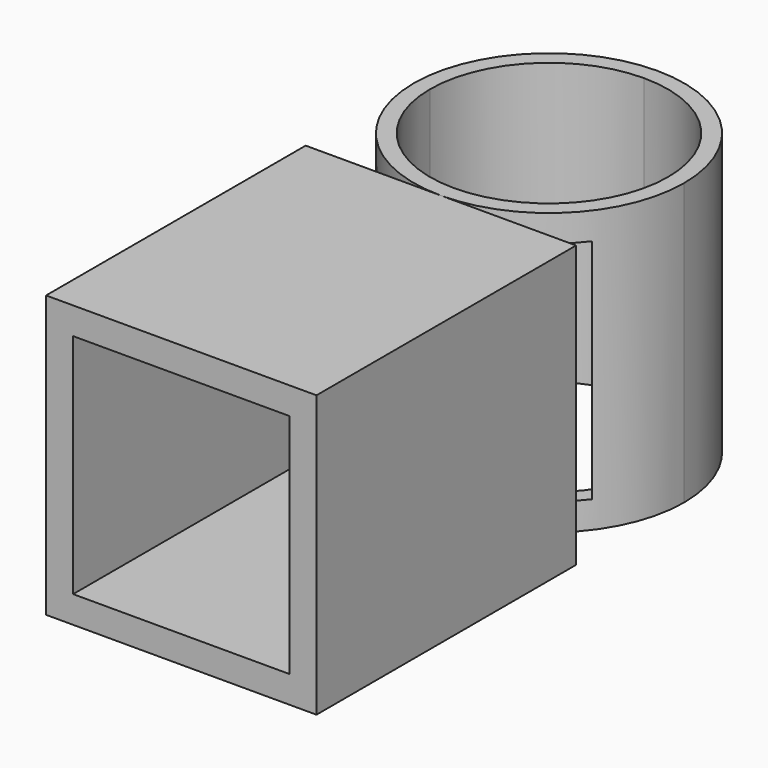
from build123d import *

# Parameters (mm, degrees)
F1_DEPTH = 26
F3_W     = 25
F3_H     = 26
F4_DEPTH = 30
F5_T     = -2.5
F6_DEPTH = 15


with BuildPart() as f1:
    # F0 (on Top) → F1 (new body)
    with BuildSketch(Plane.XY):
        with BuildLine():
            Line((11, 0), (12.5, 0))
            ThreePointArc((12.5, 0), (8.8388347648, 8.8388347648), (0, 12.5))
            Line((0, 12.5), (0, 11))
            ThreePointArc((0, 11), (7.7781745931, 7.7781745931), (11, 0))
        make_face()
        with BuildLine():
            Line((0, 11), (0, 12.5))
            ThreePointArc((0, 12.5), (-8.8388347648, 8.8388347648), (-12.5, 0))
            Line((-12.5, 0), (-11, 0))
            ThreePointArc((-11, 0), (-7.7781745931, 7.7781745931), (0, 11))
        make_face()
        with BuildLine():
            ThreePointArc((-12.5, 0), (-8.8388347648, -8.8388347648), (0, -12.5))
            Line((0, -12.5), (0, -11))
            ThreePointArc((0, -11), (-7.7781745931, -7.7781745931), (-11, 0))
            Line((-11, 0), (-12.5, 0))
        make_face()
        with BuildLine():
            ThreePointArc((0, -12.5), (8.8388347648, -8.8388347648), (12.5, 0))
            Line((12.5, 0), (11, 0))
            ThreePointArc((11, 0), (7.7781745931, -7.7781745931), (0, -11))
            Line((0, -11), (0, -12.5))
        make_face()
    extrude(amount=F1_DEPTH)


with BuildPart() as f4:
    # F3 (on offset) → F4 (new body)
    with BuildSketch(Plane.XZ.offset(12.5)):
        with Locations((-0.0008905306, 13)):
            Rectangle(F3_W, F3_H)
    extrude(amount=F4_DEPTH)

    # F5
    f5_openings = [f4.faces().sort_by_distance(p)[0] for p in [
        (-0.000891, -42.5, 13),
    ]]
    offset(amount=F5_T, openings=f5_openings)


with BuildPart() as f6_tool:
    # F6 (cut): a face of the model
    f6_faces = [f4.part.faces().sort_by_distance(p)[0] for p in [
        (-0.0008905306, -15, 13),
    ]]
    extrude(f6_faces, amount=-F6_DEPTH)


with BuildPart() as f1_1:
    add(f1.part)

    # F6: cut by f6_tool
    add(f6_tool.part, mode=Mode.SUBTRACT)


with BuildPart() as f4_1:
    add(f4.part)

    # F6: cut by f6_tool
    add(f6_tool.part, mode=Mode.SUBTRACT)


solid = Compound([f1_1.part, f4_1.part])
